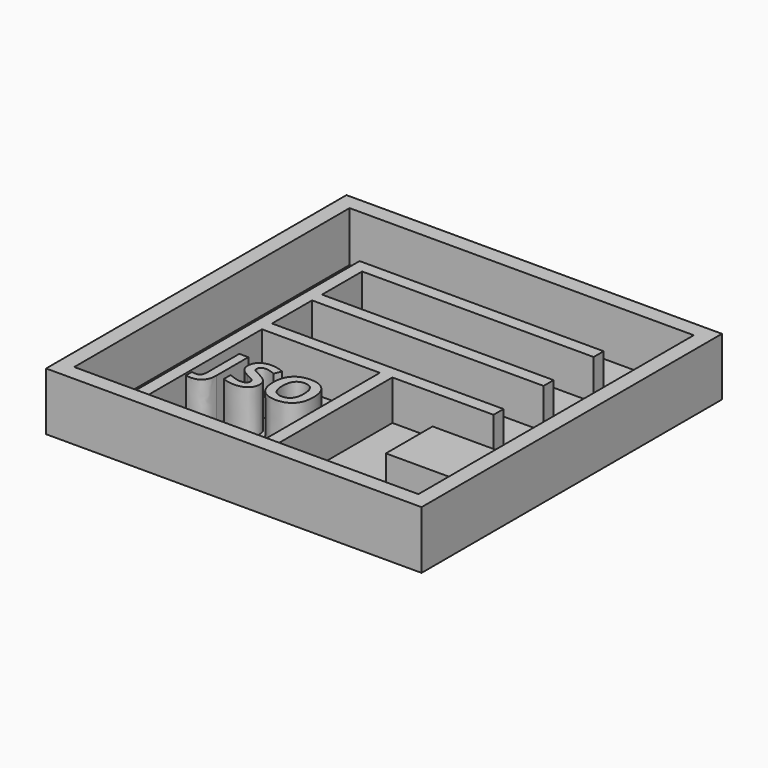
from build123d import *

# Parameters (mm, degrees)
F0_W          = 38.1
F0_H          = 38.1
F1_DEPTH      = 0.79375
F2_W          = 38.1
F2_H          = 38.1
F2_W_2        = 34.925
F2_H_2        = 34.925
F3_DEPTH      = 5.08
F5_DEPTH      = 4.064
F6_W          = 7.6031527497
F6_H          = 5.9200960677
F7_DEPTH      = 4.064
F8_R          = 1.27
F9_DEPTH      = 0.396875
F10_R         = 1.27
F11_DEPTH     = 0.396875
F12_TEXT_SIZE = 6.0453307621
F13_DEPTH     = 4.445


# Not quite as in the source:
# - Text() gives the source's letters only with a copy of the font that has no kerning and outlines rounded to 1/6400 em; it was checked with that copy


with BuildPart() as f1:
    # F0 (on Top) → F1 (new body)
    with BuildSketch(Plane.XY):
        with Locations((-4.952263087, 8.1614241723)):
            Rectangle(F0_W, F0_H)
    extrude(amount=F1_DEPTH)

    # F2 (on face) → F3 (join)
    with BuildSketch(Plane.XY.offset(0.79375)):
        with Locations((-4.952263087, 8.1614241723)):
            Rectangle(F2_W, F2_H)
        with Locations((-4.952263087, 8.1614241723)):
            Rectangle(F2_W_2, F2_H_2, mode=Mode.SUBTRACT)
    extrude(amount=F3_DEPTH)

    # F4 (on face) → F5 (join)
    with BuildSketch(Plane.XY.offset(0.79375)):
        Polygon((-17.334763087, 20.5439241723), (-17.334763087, -9.3010758277), (-16.064763087, -9.3010758277), (-16.064763087, 6.5739241723), (-4.1026365943, 6.5739241723), (-4.1026365943, -9.3010758277), (-2.8326365943, -9.3010758277), (-2.8326365943, 6.5739241723), (7.430236913, 6.5739241723), (7.430236913, 7.8439241723), (-16.064763087, 7.8439241723), (-16.064763087, 12.9239241723), (7.430236913, 12.9239241723), (7.430236913, 14.1939241723), (-16.064763087, 14.1939241723), (-16.064763087, 19.2739241723), (7.430236913, 19.2739241723), (7.430236913, 20.5439241723), (-16.064763087, 20.5439241723), align=None)
    extrude(amount=F5_DEPTH)

    # F6 (on face) → F7 (join)
    with BuildSketch(Plane.XY.offset(0.79375)):
        with Locations((8.7086605381, -0.9622668149)):
            Rectangle(F6_W, F6_H)
    extrude(amount=F7_DEPTH)

    # F8 (on face) → F9 (cut)
    with BuildSketch(Plane.XY.offset(0.79375)):
        with Locations((-19.874763087, -6.5657549419)):
            Circle(F8_R)
    extrude(amount=-F9_DEPTH, mode=Mode.SUBTRACT)

    # F10 (on face) → F11 (cut)
    with BuildSketch(Plane.XY.offset(0.79375)):
        with Locations((8.7086605381, -6.6116953382)):
            Circle(F10_R)
    extrude(amount=-F11_DEPTH, mode=Mode.SUBTRACT)

    # F12 (on face) → F13 (join)
    with BuildSketch(Plane.XY.offset(0.79375)):
        with Locations((-14.9185108021, -2.7268551057)):
            Text('JSO', F12_TEXT_SIZE, font='Open Sans', font_style=FontStyle.BOLD, text_align=(TextAlign.LEFT, TextAlign.BOTTOM))
    extrude(amount=F13_DEPTH)


solid = f1.part
